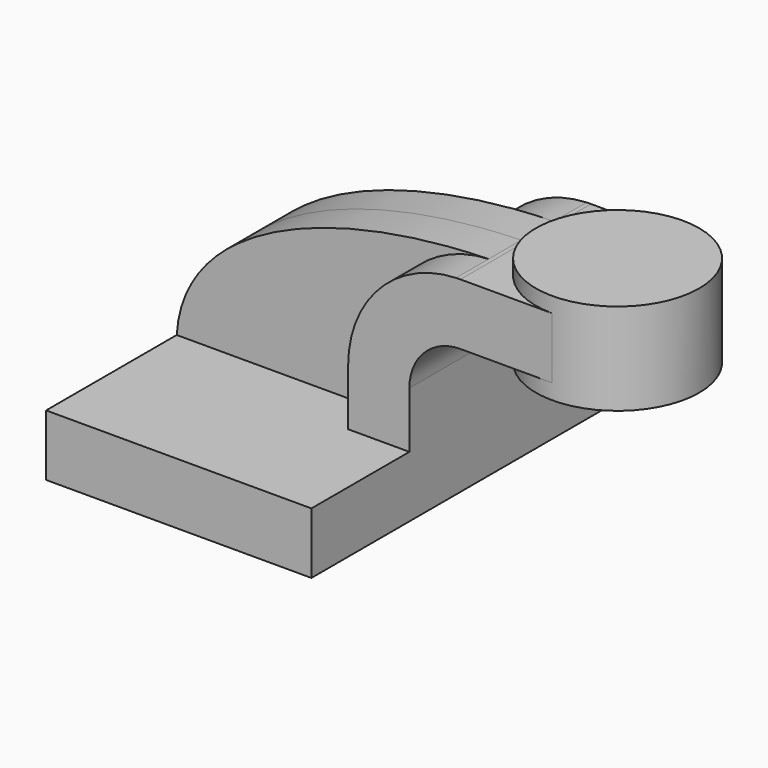
from build123d import *

# Parameters (mm, degrees)
F1_DEPTH = 63.5
F0_W     = 25.4
F0_H     = 19.05
F2_DEPTH = 25.4
F3_DEPTH = 12.7


with BuildPart() as f1:
    # F0 (on Front) → F1 (new body, symmetric)
    with BuildSketch(Plane.XZ):
        Polygon((-41.275, -9.525), (41.275, -9.525), (41.275, 9.525), (22.225, 9.525), (-41.275, 9.525), align=None)
    extrude(amount=F1_DEPTH, both=True)

    # F0 (on Front) → F2 (join, symmetric)
    with BuildSketch(Plane.XZ):
        with BuildLine():
            Line((22.225, 9.525), (41.275, 9.525))
            Line((41.275, 9.525), (41.275, 27.0002))
            ThreePointArc((41.275, 27.0002), (45.9246798487, 38.2255201513), (57.15, 42.8752))
            Line((57.15, 42.8752), (60.325, 42.8752))
            Line((60.325, 42.8752), (60.325, 61.9252))
            Line((60.325, 61.9252), (57.15, 61.9252))
            add(Edge.make_bspline(
                [(55.7747590851, 61.8981130812), (56.2330882006, 61.9086209195), (56.6915145362, 61.9176497894), (57.15, 61.9252)],
                knots=[110.4504448216, 110.4504448216, 110.4504448216, 110.4504448216, 111.5045361635, 111.5045361635, 111.5045361635, 111.5045361635], degree=3))
            ThreePointArc((55.7747590851, 61.8981130812), (31.9727690765, 51.2048001418), (22.225, 27.0002))
            Line((22.225, 27.0002), (22.225, 9.525))
        make_face()
        with Locations((73.025, 52.4002)):
            Rectangle(F0_W, F0_H)
    extrude(amount=F2_DEPTH, both=True)

    # F0 (on Front) → F3 (join, symmetric)
    with BuildSketch(Plane.XZ):
        with BuildLine():
            add(Edge.make_bspline(
                [(-41.275, 9.525), (-39.2076677015, 43.4578572164), (7.7498368859, 60.7970743394), (55.7747590851, 61.8981130812)],
                knots=[0, 0, 0, 0, 110.4504448216, 110.4504448216, 110.4504448216, 110.4504448216], degree=3))
            Line((-41.275, 9.525), (22.225, 9.525))
            Line((22.225, 9.525), (22.225, 27.0002))
            ThreePointArc((22.225, 27.0002), (31.9727690765, 51.2048001418), (55.7747590851, 61.8981130812))
        make_face()
    extrude(amount=F3_DEPTH, both=True)

    # F0 (on Front) → F4 (revolve)
    with BuildSketch(Plane.XZ):
        Polygon((85.725, 61.9252), (85.725, 42.8752), (85.725, 38.1), (111.125, 38.1), (111.125, 66.675), (85.725, 66.675), align=None)
    revolve(axis=Axis((85.725, 0, 52.3875), (0, 0, 1)))


solid = f1.part
